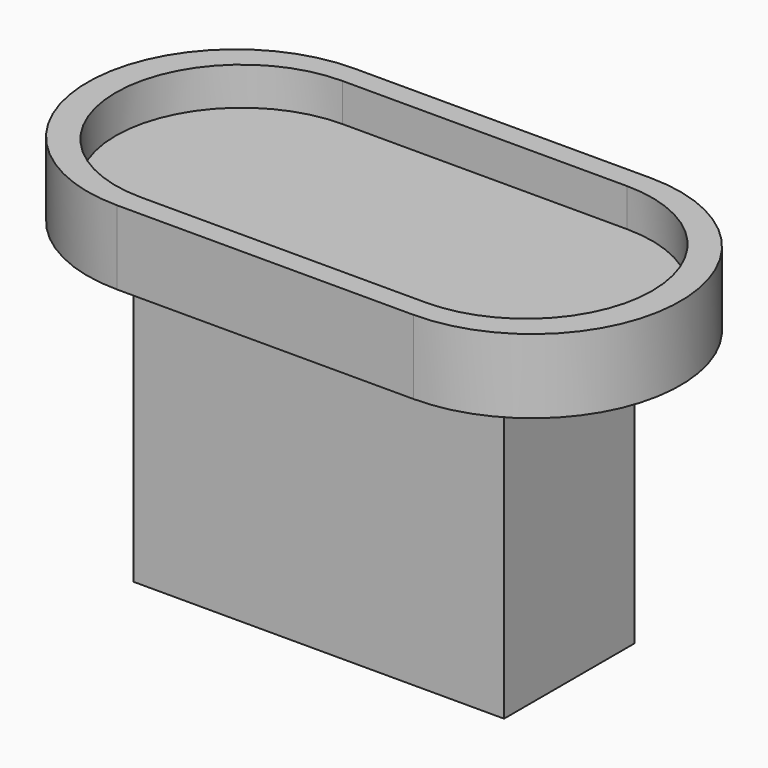
from build123d import *

# Parameters (mm, degrees)
F1_DEPTH = 6.35
F2_W     = 31.75
F2_H     = 13.97
F3_DEPTH = 25.4
F5_DEPTH = 3.2512


# Not quite as in the source:
# - a feature names something its author has since deleted; it is built from what else it names


with BuildPart() as f1:
    # F0 (on Top) → F1 (new body)
    with BuildSketch(Plane.XY):
        with BuildLine():
            Line((-12.7, -12.7), (12.7, -12.7))
            ThreePointArc((12.7, -12.7), (25.4, 0), (12.7, 12.7))
            Line((12.7, 12.7), (-12.7, 12.7))
            ThreePointArc((-12.7, 12.7), (-25.4, 0), (-12.7, -12.7))
        make_face()
    extrude(amount=F1_DEPTH)

    # F2 (on face) → F3 (join)
    with BuildSketch(Plane(origin=(0, 0, 0), x_dir=(1, 0, 0), z_dir=(0, 0, -1))):
        Rectangle(F2_W, F2_H)
    extrude(amount=F3_DEPTH)

    # F4 (on face) → F5 (cut)
    with BuildSketch(Plane.XY.offset(6.35)):
        with BuildLine():
            Line((-12.192, -10.795), (12.192, -10.795))
            ThreePointArc((12.192, -10.795), (22.987, 0), (12.192, 10.795))
            Line((12.192, 10.795), (-12.192, 10.795))
            ThreePointArc((-12.192, 10.795), (-22.987, 0), (-12.192, -10.795))
        make_face()
    extrude(amount=-F5_DEPTH, mode=Mode.SUBTRACT)


solid = f1.part
